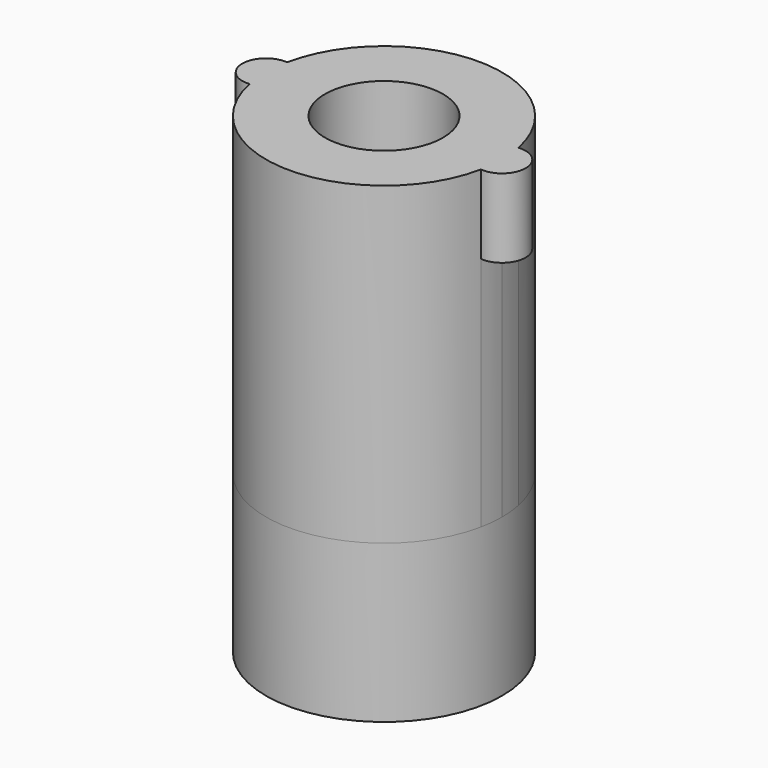
from build123d import *
from build123d import SkipClean  # not in build123d's __all__

# Parameters (mm, degrees)
F0_R     = 7.5
F1_DEPTH = 40
F2_START = 30
F2_DEPTH = 10
F3_R     = 15
F4_DEPTH = 20
F6_D     = 4.4
F6_DEPTH = 19
F6_TIP   = 1.3218933619


# Not quite as in the source:
# - after a boolean that leaves OpenCascade's solid faulty, fix() repairs it


with BuildPart() as f1:
    # F0 (on Top) → F1 (new body)
    with BuildSketch(Plane.XY):
        with BuildLine():
            ThreePointArc((14.7, -2.9849623113), (14.9248115566, -1.5), (15, 0))
            ThreePointArc((15, 0), (14.9248115566, 1.5), (14.7, 2.9849623113))
            ThreePointArc((14.7, 2.9849623113), (0, 15), (-14.7, 2.9849623113))
            ThreePointArc((-14.7, 2.9849623113), (-15, 0), (-14.7, -2.9849623113))
            ThreePointArc((-14.7, -2.9849623113), (0, -15), (14.7, -2.9849623113))
        make_face()
        Circle(F0_R, mode=Mode.SUBTRACT)
    extrude(amount=F1_DEPTH)

    # F0 (on Top) → F2 (join)
    with BuildSketch(Plane.XY.offset(F2_START)):
        with BuildLine():
            ThreePointArc((-14.7, -2.9849623113), (-15, 0), (-14.7, 2.9849623113))
            ThreePointArc((-14.7, 2.9849623113), (-18, 0), (-14.7, -2.9849623113))
        make_face()
        with BuildLine():
            ThreePointArc((14.7, 2.9849623113), (14.9248115566, 1.5), (15, 0))
            ThreePointArc((15, 0), (14.9248115566, -1.5), (14.7, -2.9849623113))
            ThreePointArc((14.7, -2.9849623113), (18, 0), (14.7, 2.9849623113))
        make_face()
    extrude(amount=F2_DEPTH)

    # F3 (on face) → F4 (join)
    with BuildSketch(Plane(origin=(0, 0, 0), x_dir=(1, 0, 0), z_dir=(0, 0, -1))):
        Circle(F3_R)
    with SkipClean():  # cleaning this boolean's faces spoils the solid; the shape is the same uncleaned
        extrude(amount=F4_DEPTH)

    # F6
    with Locations(Plane(origin=(0, 0, -20), x_dir=(1, 0, 0), z_dir=(0, 0, -1))):
        with Locations((0, 0)):
            Hole(F6_D / 2, depth=F6_DEPTH)
            with Locations((0, 0, -(F6_DEPTH + F6_TIP / 2))):  # 118° drill point
                Cone(0, F6_D / 2, F6_TIP, mode=Mode.SUBTRACT)

    add(f1.part.fix(), mode=Mode.REPLACE)


solid = f1.part
